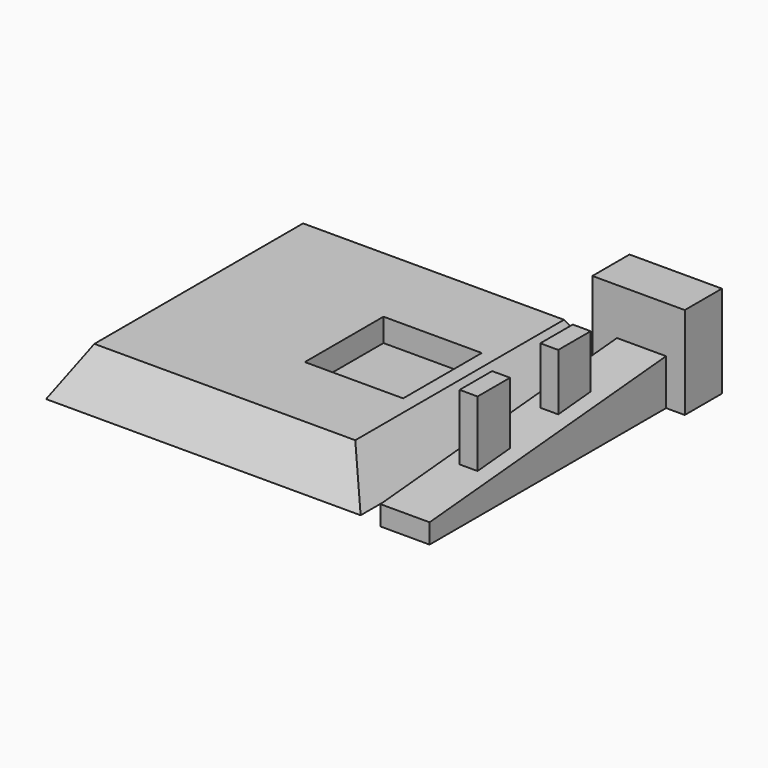
from build123d import *

# Parameters (mm, degrees)
F0_W          = 40.64
F0_H          = 40.64
F1_DEPTH      = 6
F1_TAPER      = 30
F2_W          = 12.7
F2_H          = 12.7000013893
F3_DEPTH      = 25.4
F3_DEPTH_BACK = 3
F4_W          = 11.938
F4_H          = 11.938
F5_DEPTH      = 6
F6_W          = 6.35
F6_H          = 6.35
F7_DEPTH      = 44.196
F8_T4_DEPTH   = 230.8538605698
F10_START     = 0.3048
F9_W          = 2.3218709975
F9_H          = 5.2457088605
F10_DEPTH     = 11.9356720546


# Not quite as in the source:
# - a fillet or chamfer that OpenCascade refuses, or shapes differently, is made with other operations: its cross-section is extruded or revolved along the edge and cut away or added


with BuildPart() as f1:
    # F0 (on Top) → F1 (new body)
    with BuildSketch(Plane.XY):
        with Locations((-20.32, 14.8309261845)):
            Rectangle(F0_W, F0_H)
    extrude(amount=F1_DEPTH, taper=F1_TAPER)

    # F2 (on face) → F3 (cut, two sides)
    with BuildSketch(Plane.XY.offset(6)) as f3_sk:
        with Locations((-11.7568750866, 14.4863990135)):
            Rectangle(F2_W, F2_H)
    extrude(amount=F3_DEPTH, mode=Mode.SUBTRACT)
    extrude(f3_sk.sketch, amount=-F3_DEPTH_BACK, mode=Mode.SUBTRACT)


with BuildPart() as f5:
    # F4 (on Front) → F5 (new body)
    with BuildSketch(Plane.XZ):
        with Locations((31.3934258791, 6.2714720546)):
            Rectangle(F4_W, F4_H)
    extrude(amount=F5_DEPTH)

    # F6 (on Front) → F7 (join)
    with BuildSketch(Plane.XZ):
        with Locations((31.77456907, 3.4775143722)):
            Rectangle(F6_W, F6_H)
    extrude(amount=F7_DEPTH)

    # F8: chamfer of 43.18 x 3.81 on 1 edges, made by hand


with BuildPart() as f8_tool2:
    # F8_s3 → F8_t4 (new body)
    with BuildSketch(Plane.YZ.offset(147.2014993549)):
        Polygon((-1.016, 6.6525143722), (-44.196, 2.8425143722), (-44.196, 6.6525143722), align=None)
    extrude(amount=-F8_T4_DEPTH)

    split(bisect_by=Plane.XZ.offset(6), keep=Keep.TOP)


with BuildPart() as f5_1:
    add(f5.part)

    # F8_t1: cut F8_tool2
    add(f8_tool2.part, mode=Mode.SUBTRACT)

    # F9 (on Top) → F10 (join)
    with BuildSketch(Plane.XY.offset(F10_START)):
        with Locations((31.6735515371, -31.1798783951)):
            Rectangle(F9_W, F9_H)
        with Locations((31.6735515371, -18.1505319482)):
            Rectangle(F9_W, F9_H)
    extrude(amount=F10_DEPTH)


with BuildPart() as f5_2:
    # F11: moved
    add(f5_1.part.moved(Location((-25.146, 37.592, 0))))


solid = Compound([f1.part, f5_2.part])
